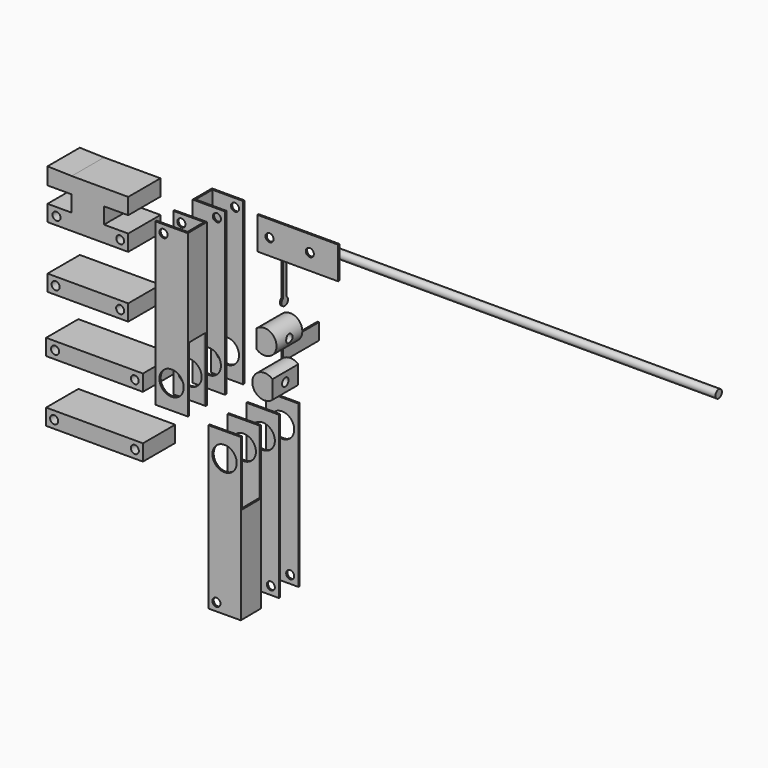
from build123d import *

# Parameters (mm, degrees)
F1_DEPTH  = 100
F2_R      = 7.5
F2_R_2    = 2.5
F3_DEPTH  = 15.001
F4_W      = 13
F4_H      = 40
F5_DEPTH  = 20.1627097718
F6_DEPTH  = 100
F7_R      = 7.5
F7_R_2    = 2.5
F8_DEPTH  = 16.001
F9_W      = 14
F9_H      = 40
F10_DEPTH = 20.1691592966
F11_W     = 50
F11_H     = 20
F11_R     = 2.5
F12_DEPTH = 1
F13_R     = 2.5
F13_R_2   = 7.5
F14_DEPTH = 45.1330833913
F15_R     = 7.5
F15_R_2   = 2.5
F16_DEPTH = 46.1330833913
F17_W     = 14
F17_H     = 40
F18_DEPTH = 53.5847666336
F19_W     = 13
F19_H     = 40
F20_DEPTH = 25
F22_DEPTH = 20
F23_R     = 2.5
F24_DEPTH = 250
F25_W     = 50
F25_H     = 10
F25_R     = 2.5
F26_DEPTH = 25
F25_R_2   = 2.4144593705
F25_W_2   = 60
F27_DEPTH = 25
F28_R     = 2.5
F29_DEPTH = 136.2251037518
F30_R     = 2.5
F31_DEPTH = 214.5146418358
F33_DEPTH = 1
F34_W     = 1
F34_H     = 10
F35_DEPTH = 25


# Not quite as in the source:
# - a feature names something its author has since deleted; it is built from what else it names


with BuildPart() as f1:
    # F0 (on Top) → F1 (new body)
    with BuildSketch(Plane.XY):
        Polygon((0, 14), (0, 15), (-20, 15), (-20, 0), (0, 0), (0, 1), (-19, 1), (-19, 14), align=None)
    extrude(amount=F1_DEPTH)

    # F2 (on face) → F3 (cut, through all)
    with BuildSketch(Plane.XZ):
        with Locations((-10, 15)):
            Circle(F2_R)
        with Locations((-5, 95)):
            Circle(F2_R_2)
    extrude(amount=-F3_DEPTH, mode=Mode.SUBTRACT)

    # F4 (on face) → F5 (cut, through all)
    with BuildSketch(Plane(origin=(-20, 0, 0), x_dir=(0, -1, 0), z_dir=(-1, 0, 0))):
        with Locations((-7.5, 20)):
            Rectangle(F4_W, F4_H)
    extrude(amount=-F5_DEPTH, mode=Mode.SUBTRACT)


with BuildPart() as f1b:
    # F0 (on Top) → F1, piece 2 (new body)
    with BuildSketch(Plane.XY):
        Polygon((0.051417134, -13.985459061), (-19.9480422158, -14.1325159114), (-19.9406893732, -15.1324888789), (-0.941202991, -14.992784871), (-0.8456160382, -27.9924334484), (-19.837749578, -28.1320833905), (-19.837749578, -29.1321104238), (0.1617097718, -28.9850535734), align=None)
    extrude(amount=F1_DEPTH)

    # F13 (on face) → F14 (cut, through all)
    with BuildSketch(Plane(origin=(0.2131255159, -28.9846755113, 0), x_dir=(0.9999729675, 0.0073528425, 0), z_dir=(0.0073528425, -0.9999729675, 0))):
        with Locations((-15.051417134, 95)):
            Circle(F13_R)
        with Locations((-10.051417134, 15)):
            Circle(F13_R_2)
    extrude(amount=-F14_DEPTH, mode=Mode.SUBTRACT)

    # F19 (on face) → F20 (cut)
    with BuildSketch(Plane(origin=(-0.0514157441, -0.0003780621, 0), x_dir=(-0.0073528425, 0.9999729675, 0), z_dir=(0.9999729675, 0.0073528425, 0))):
        with Locations((-21.485459061, 20)):
            Rectangle(F19_W, F19_H)
    extrude(amount=-F20_DEPTH, mode=Mode.SUBTRACT)


with BuildPart() as f6:
    # F0 (on Top) → F6 (new body)
    with BuildSketch(Plane.XY):
        Polygon((33.4159745649, 0), (33.4159745649, 1), (14.4159745649, 1), (14.4159745649, 15), (33.4159745649, 15), (33.4159745649, 16), (13.4159745649, 16), (13.4159745649, 0), align=None)
    extrude(amount=-F6_DEPTH)

    # F7 (on face) → F8 (cut, through all)
    with BuildSketch(Plane.XZ):
        with Locations((23.4159745649, -15)):
            Circle(F7_R)
        with Locations((28.4159745649, -95)):
            Circle(F7_R_2)
    extrude(amount=-F8_DEPTH, mode=Mode.SUBTRACT)

    # F9 (on face) → F10 (cut, through all)
    with BuildSketch(Plane(origin=(13.4159745649, 0, 0), x_dir=(0, -1, 0), z_dir=(-1, 0, 0))):
        with Locations((-8, -20)):
            Rectangle(F9_W, F9_H)
    extrude(amount=-F10_DEPTH, mode=Mode.SUBTRACT)


with BuildPart() as f6b:
    # F0 (on Top) → F6, piece 2 (new body)
    with BuildSketch(Plane.XY):
        Polygon((33.4664883811, -13.7397566624), (13.4670290313, -13.8868135128), (13.4743818739, -14.8867864803), (32.4738682561, -14.7470824724), (32.5768080514, -28.7467040172), (13.5846745117, -28.8863539594), (13.5846745117, -29.8863809926), (33.5841338614, -29.7393241422), align=None)
    extrude(amount=-F6_DEPTH)

    # F15 (on face) → F16 (cut, through all)
    with BuildSketch(Plane(origin=(0.2204783584, -29.9846484788, 0), x_dir=(0.9999729675, 0.0073528425, 0), z_dir=(0.0073528425, -0.9999729675, 0))):
        with Locations((23.3645574309, -15)):
            Circle(F15_R)
        with Locations((18.3645574309, -95)):
            Circle(F15_R_2)
    extrude(amount=-F16_DEPTH, mode=Mode.SUBTRACT)

    # F17 (on face) → F18 (cut, through all)
    with BuildSketch(Plane(origin=(33.3636555031, 0.2453243365, 0), x_dir=(-0.0073528425, 0.9999729675, 0), z_dir=(0.9999729675, 0.0073528425, 0))):
        with Locations((-21.985459061, -20)):
            Rectangle(F17_W, F17_H)
    extrude(amount=-F18_DEPTH, mode=Mode.SUBTRACT)


with BuildPart() as f12:
    # F11 (on Front) → F12 (new body)
    with BuildSketch(Plane.XZ):
        with Locations((45.8931141218, 95.3558683395)):
            Rectangle(F11_W, F11_H)
        with Locations((28.3931141218, 95.3558683395)):
            Circle(F11_R, mode=Mode.SUBTRACT)
        with Locations((53.3931141218, 95.3558683395)):
            Circle(F11_R, mode=Mode.SUBTRACT)
    extrude(amount=F12_DEPTH)


with BuildPart() as f22:
    # F21 (on Front) → F22 (new body)
    with BuildSketch(Plane.XZ):
        with BuildLine():
            Line((35.4863581642, 55.8813297105), (35.4863581642, 44.6073331245))
            ThreePointArc((35.4863581642, 44.6073331245), (47.9335038306, 50.2443314175), (35.4863581642, 55.8813297105))
        make_face()
    extrude(amount=F22_DEPTH)

    # F30 (on face) → F31 (cut, through all)
    with BuildSketch(Plane(origin=(35.4863581642, 0, 0), x_dir=(0, -1, 0), z_dir=(-1, 0, 0))):
        with Locations((10, 50.2443314175)):
            Circle(F30_R)
    extrude(amount=-F31_DEPTH, mode=Mode.SUBTRACT)


with BuildPart() as f22b:
    # F21 (on Front) → F22, piece 2 (new body)
    with BuildSketch(Plane.XZ):
        with BuildLine():
            Line((45.380649497, 20.1312099156), (45.380649497, 31.4052065016))
            ThreePointArc((45.380649497, 31.4052065016), (32.9335038306, 25.7682082086), (45.380649497, 20.1312099156))
        make_face()
    extrude(amount=F22_DEPTH)

    # F28 (on face) → F29 (cut, through all)
    with BuildSketch(Plane.YZ.offset(45.380649497)):
        with Locations((-10, 25.7682082086)):
            Circle(F28_R)
    extrude(amount=-F29_DEPTH, mode=Mode.SUBTRACT)


with BuildPart() as f24:
    # F23 (on Right) → F24 (new body)
    with BuildSketch(Plane.YZ):
        with Locations((69.883659482, 53.4276850522)):
            Circle(F23_R)
    extrude(amount=F24_DEPTH)


with BuildPart() as f26:
    # F25 (on Front) → F26 (new body)
    with BuildSketch(Plane.XZ):
        with Locations((-64.9493469292, 42.0624911785)):
            Rectangle(F25_W, F25_H)
        with Locations((-84.9493469292, 42.0624911785)):
            Circle(F25_R, mode=Mode.SUBTRACT)
        with Locations((-44.9493469292, 42.0624911785)):
            Circle(F25_R, mode=Mode.SUBTRACT)
    extrude(amount=F26_DEPTH)


with BuildPart() as f26b:
    # F25 (on Front) → F26, piece 2 (new body)
    with BuildSketch(Plane.XZ):
        Polygon((-89.9493469292, 85.124527216), (-89.9493469292, 75.124527216), (-39.9493469292, 75.124527216), (-39.9493469292, 85.124527216), (-54.9493469292, 85.124527216), (-54.9493469292, 95.124527216), (-39.9493469292, 95.124527216), (-39.9493469292, 105.124527216), (-54.9493469292, 105.124527216), (-64.9493469292, 105.124527216), (-74.9493469292, 105.124527216), (-89.9493469292, 105.5638343096), (-89.9493469292, 95.124527216), (-74.9493469292, 95.124527216), (-74.9493469292, 85.124527216), align=None)
        with Locations((-84.3778774142, 80.124527216)):
            Circle(F25_R, mode=Mode.SUBTRACT)
        with Locations((-44.9493469292, 80.124527216)):
            Circle(F25_R_2, mode=Mode.SUBTRACT)
    extrude(amount=F26_DEPTH)


with BuildPart() as f27:
    # F25 (on Front) → F27 (new body)
    with BuildSketch(Plane.XZ):
        with Locations((-60.8434542548, -31.3186603598)):
            Rectangle(F25_W_2, F25_H)
        with Locations((-85.8434542548, -31.3186603598)):
            Circle(F25_R, mode=Mode.SUBTRACT)
        with Locations((-35.8434542548, -31.3186603598)):
            Circle(F25_R, mode=Mode.SUBTRACT)
    extrude(amount=F27_DEPTH)


with BuildPart() as f27b:
    # F25 (on Front) → F27, piece 2 (new body)
    with BuildSketch(Plane.XZ):
        with Locations((-60.8434542548, 6.7433756776)):
            Rectangle(F25_W_2, F25_H)
        with Locations((-85.2719847398, 6.7433756776)):
            Circle(F25_R, mode=Mode.SUBTRACT)
        with Locations((-35.8434542548, 6.7433756776)):
            Circle(F25_R_2, mode=Mode.SUBTRACT)
    extrude(amount=F27_DEPTH)


with BuildPart() as f33:
    # F32 (on Right) → F33 (new body)
    with BuildSketch(Plane.YZ):
        with BuildLine():
            Line((47.762863338, 8.6800148711), (47.762863338, 20.4667558931))
            ThreePointArc((47.762863338, 20.4667558931), (46.3052242994, 24.9978365004), (44.8475852609, 20.4667558931))
            Line((44.8475852609, 20.4667558931), (44.8475852609, 8.6800148711))
            Line((44.8475852609, 8.6800148711), (44.8475852609, 0))
            Line((44.8475852609, 0), (47.762863338, 0))
            Line((47.762863338, 0), (47.762863338, 8.6800148711))
        make_face()
    extrude(amount=-F33_DEPTH)

    # F34 (on face) → F35 (join)
    with BuildSketch(Plane(origin=(0, 47.762863338, 0), x_dir=(-1, 0, 0), z_dir=(0, 1, 0))):
        with Locations((0.5, 5)):
            Rectangle(F34_W, F34_H)
    extrude(amount=F35_DEPTH)


with BuildPart() as f33b:
    # F32 (on Right) → F33, piece 2 (new body)
    with BuildSketch(Plane.YZ):
        with BuildLine():
            ThreePointArc((44.8475852609, 34.1576339639), (46.3052242994, 29.6265533566), (47.762863338, 34.1576339639))
            Line((47.762863338, 34.1576339639), (47.762863338, 45.944374986))
            Line((47.762863338, 45.944374986), (47.762863338, 54.6243898571))
            Line((47.762863338, 54.6243898571), (44.8475852609, 54.6243898571))
            Line((44.8475852609, 54.6243898571), (44.8475852609, 45.944374986))
            Line((44.8475852609, 45.944374986), (44.8475852609, 34.1576339639))
        make_face()
    extrude(amount=-F33_DEPTH)


solid = Compound([f1.part, f1b.part, f6.part, f6b.part, f12.part, f22.part, f22b.part, f24.part, f26.part, f26b.part, f27.part, f27b.part, f33.part, f33b.part])
